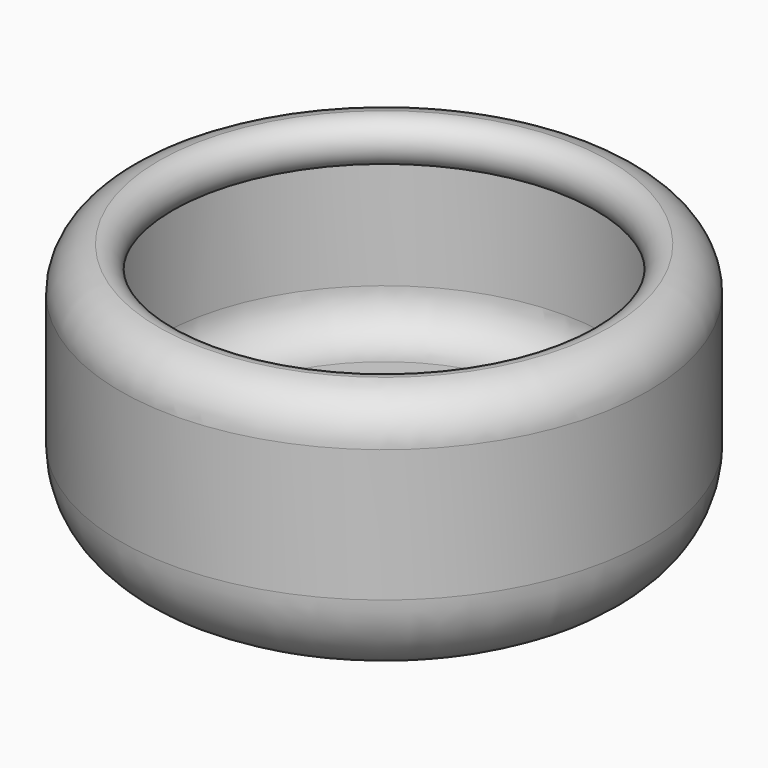
from build123d import *

# Parameters (mm, degrees)
F0_R     = 5.125
F1_DEPTH = 1.5
F0_R_2   = 6
F2_DEPTH = 6
F3_R     = 2


# Not quite as in the source:
# - a fillet or chamfer that OpenCascade refuses, or shapes differently, is made with other operations: its cross-section is extruded or revolved along the edge and cut away or added


with BuildPart() as f1:
    # F0 (on Top) → F1 (new body)
    with BuildSketch(Plane.XY):
        Circle(F0_R)
    extrude(amount=F1_DEPTH)

    # F0 (on Top) → F2 (join)
    with BuildSketch(Plane.XY):
        Circle(F0_R_2)
        Circle(F0_R, mode=Mode.SUBTRACT)
    extrude(amount=F2_DEPTH)

    # F3
    f3_edges = [f1.edges().sort_by_distance(p)[0] for p in [
        (-6, 0, 0),
    ]]
    fillet(f3_edges, radius=F3_R)

    # F4 (on Right) → F5 (revolve)
    with BuildSketch(Plane.YZ):
        with BuildLine():
            Line((-5.125, 6), (-5.125, 5))
            ThreePointArc((-5.125, 5), (-4.625, 5.5), (-5.125, 6))
        make_face()
    revolve(axis=Axis((0, 0, 6), (0, 0, 1)))

    # F6: fillet of radius 1 on 2 edges, made by hand

    # F6_s1 → F6_t2 (revolve)
    with BuildSketch(Plane.XZ):
        with BuildLine():
            ThreePointArc((5.125, 2.5), (4.8321067812, 1.7928932188), (4.125, 1.5))
            Line((4.125, 1.5), (5.125, 1.5))
            Line((5.125, 1.5), (5.125, 2.5))
        make_face()
    revolve(axis=Axis((0, 0, 1.5), (0, 0, 1)))

    # F6_s3 → F6_t4 (revolve, cut)
    with BuildSketch(Plane.XZ):
        with BuildLine():
            ThreePointArc((6, 5.0078432584), (5.75, 5.6692810861), (5.125, 6))
            Line((5.125, 6), (6, 6))
            Line((6, 6), (6, 5.0078432584))
        make_face()
    revolve(axis=Axis((0, 0, 6), (0, 0, 1)), mode=Mode.SUBTRACT)


solid = f1.part
